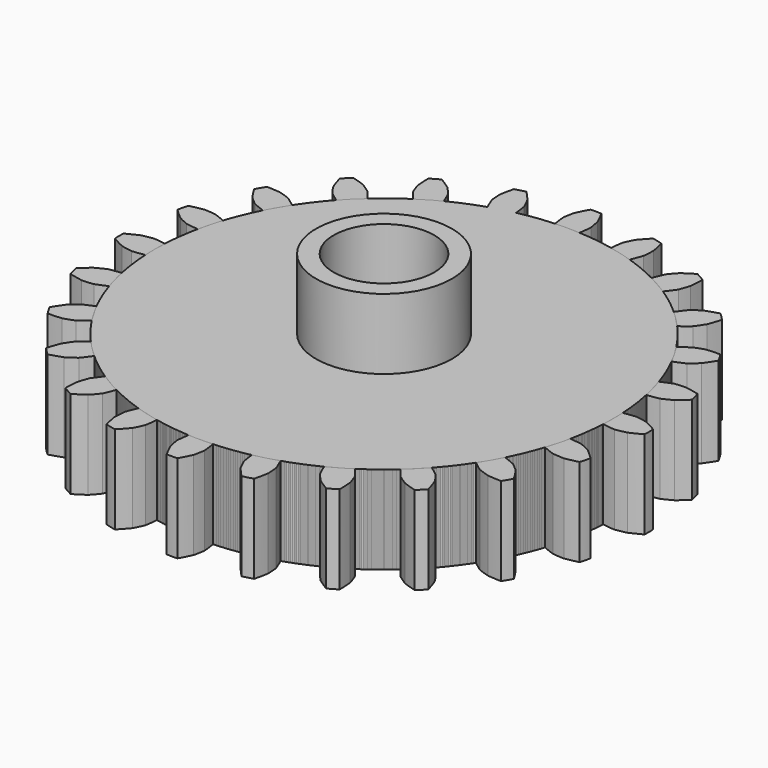
from build123d import *

# Parameters (mm, degrees)
F1_DEPTH = 5
F2_COUNT = 24
F3_R     = 2.85
F4_DEPTH = 25
F5_R     = 3.85
F5_R_2   = 2.85
F6_DEPTH = 4


# Not quite as in the source:
# - a feature of the source that left no trace in its solid (it failed there, or was rolled back) is left out


with BuildPart() as f1:
    # F0 (on Top) → F1 (new body)
    with BuildSketch(Plane.XY):
        with BuildLine():
            ThreePointArc((-0.6884619994, 12.9817572029), (-8.9456691759, -9.4326562005), (13, 0))
            ThreePointArc((13, 0), (9.4359199575, 8.9422264876), (0.6979362223, 12.9812512891))
            Line((0.6979362223, 12.9812512891), (0.6595878513, 12.8166601062))
            Line((0.6595878513, 12.8166601062), (-0.6884619994, 12.8166601062))
            Line((-0.6884619994, 12.8166601062), (-0.6884619994, 12.9817572029))
        make_face()
        with BuildLine():
            Line((0.6595878513, 12.8166601062), (0.6979362223, 12.9812512891))
            ThreePointArc((0.6979362223, 12.9812512891), (0.0047438605, 12.9999991345), (-0.6884619994, 12.9817572029))
            Line((-0.6884619994, 12.9817572029), (-0.6884619994, 12.8166601062))
            Line((-0.6884619994, 12.8166601062), (0.6595878513, 12.8166601062))
        make_face()
        with BuildLine():
            ThreePointArc((-0.6884619994, 12.9817572029), (0.0047438605, 12.9999991345), (0.6979362223, 12.9812512891))
            Line((0.6979362223, 12.9812512891), (0.7013501859, 12.9959040186))
            ThreePointArc((0.7013501859, 12.9959040186), (0.7485258682, 13.3381143086), (0.7812866085, 13.6820040604))
            ThreePointArc((0.7812866085, 13.6820040604), (0.7246476562, 14.0030111675), (0.6551136173, 14.3214739615))
            ThreePointArc((0.6551136173, 14.3214739615), (0.4878270863, 14.6723504286), (0.3076734335, 15.0167974346))
            ThreePointArc((0.3076734335, 15.0167974346), (0.0022476478, 15.0264990738), (-0.3031776772, 15.0167829421))
            ThreePointArc((-0.3031776772, 15.0167829421), (-0.4904903849, 14.6709788581), (-0.6630231094, 14.3175683689))
            ThreePointArc((-0.6630231094, 14.3175683689), (-0.7323663603, 14.0016121807), (-0.7822406896, 13.6820040604))
            ThreePointArc((-0.7822406896, 13.6820040604), (-0.7420135102, 13.3383984362), (-0.6884619994, 12.9966159225))
            Line((-0.6884619994, 12.9966159225), (-0.6884619994, 12.9817572029))
        make_face()
    extrude(amount=F1_DEPTH)


with BuildPart() as f2_1:
    # F2: instance of F1
    add(f1.part.rotate(Axis((0, 0, 0), (0, 0, -1)), 1 * 360 / F2_COUNT))


with BuildPart() as f2_2:
    # F2: instance of F1
    add(f1.part.rotate(Axis((0, 0, 0), (0, 0, -1)), 2 * 360 / F2_COUNT))


with BuildPart() as f2_3:
    # F2: instance of F1
    add(f1.part.rotate(Axis((0, 0, 0), (0, 0, -1)), 3 * 360 / F2_COUNT))


with BuildPart() as f2_4:
    # F2: instance of F1
    add(f1.part.rotate(Axis((0, 0, 0), (0, 0, -1)), 4 * 360 / F2_COUNT))


with BuildPart() as f2_5:
    # F2: instance of F1
    add(f1.part.rotate(Axis((0, 0, 0), (0, 0, -1)), 5 * 360 / F2_COUNT))


with BuildPart() as f2_6:
    # F2: instance of F1
    add(f1.part.rotate(Axis((0, 0, 0), (0, 0, -1)), 6 * 360 / F2_COUNT))


with BuildPart() as f2_7:
    # F2: instance of F1
    add(f1.part.rotate(Axis((0, 0, 0), (0, 0, -1)), 7 * 360 / F2_COUNT))


with BuildPart() as f2_8:
    # F2: instance of F1
    add(f1.part.rotate(Axis((0, 0, 0), (0, 0, -1)), 8 * 360 / F2_COUNT))


with BuildPart() as f2_9:
    # F2: instance of F1
    add(f1.part.rotate(Axis((0, 0, 0), (0, 0, -1)), 9 * 360 / F2_COUNT))


with BuildPart() as f2_10:
    # F2: instance of F1
    add(f1.part.rotate(Axis((0, 0, 0), (0, 0, -1)), 10 * 360 / F2_COUNT))


with BuildPart() as f2_11:
    # F2: instance of F1
    add(f1.part.rotate(Axis((0, 0, 0), (0, 0, -1)), 11 * 360 / F2_COUNT))


with BuildPart() as f2_12:
    # F2: instance of F1
    add(f1.part.rotate(Axis((0, 0, 0), (0, 0, -1)), 12 * 360 / F2_COUNT))


with BuildPart() as f2_13:
    # F2: instance of F1
    add(f1.part.rotate(Axis((0, 0, 0), (0, 0, -1)), 13 * 360 / F2_COUNT))


with BuildPart() as f2_14:
    # F2: instance of F1
    add(f1.part.rotate(Axis((0, 0, 0), (0, 0, -1)), 14 * 360 / F2_COUNT))


with BuildPart() as f2_15:
    # F2: instance of F1
    add(f1.part.rotate(Axis((0, 0, 0), (0, 0, -1)), 15 * 360 / F2_COUNT))


with BuildPart() as f2_16:
    # F2: instance of F1
    add(f1.part.rotate(Axis((0, 0, 0), (0, 0, -1)), 16 * 360 / F2_COUNT))


with BuildPart() as f2_17:
    # F2: instance of F1
    add(f1.part.rotate(Axis((0, 0, 0), (0, 0, -1)), 17 * 360 / F2_COUNT))


with BuildPart() as f2_18:
    # F2: instance of F1
    add(f1.part.rotate(Axis((0, 0, 0), (0, 0, -1)), 18 * 360 / F2_COUNT))


with BuildPart() as f2_19:
    # F2: instance of F1
    add(f1.part.rotate(Axis((0, 0, 0), (0, 0, -1)), 19 * 360 / F2_COUNT))


with BuildPart() as f2_20:
    # F2: instance of F1
    add(f1.part.rotate(Axis((0, 0, 0), (0, 0, -1)), 20 * 360 / F2_COUNT))


with BuildPart() as f2_21:
    # F2: instance of F1
    add(f1.part.rotate(Axis((0, 0, 0), (0, 0, -1)), 21 * 360 / F2_COUNT))


with BuildPart() as f2_22:
    # F2: instance of F1
    add(f1.part.rotate(Axis((0, 0, 0), (0, 0, -1)), 22 * 360 / F2_COUNT))


with BuildPart() as f2_23:
    # F2: instance of F1
    add(f1.part.rotate(Axis((0, 0, 0), (0, 0, -1)), 23 * 360 / F2_COUNT))


with BuildPart() as f4_tool:
    # F3 (on face) → F4 (new body)
    with BuildSketch(Plane.XY.offset(5)):
        Circle(F3_R)
    extrude(amount=-F4_DEPTH)


with BuildPart() as f1_1:
    add(f1.part)

    # F4: cut by f4_tool
    add(f4_tool.part, mode=Mode.SUBTRACT)


with BuildPart() as f2_1_1:
    add(f2_1.part)

    # F4: cut by f4_tool
    add(f4_tool.part, mode=Mode.SUBTRACT)


with BuildPart() as f2_2_1:
    add(f2_2.part)

    # F4: cut by f4_tool
    add(f4_tool.part, mode=Mode.SUBTRACT)


with BuildPart() as f2_3_1:
    add(f2_3.part)

    # F4: cut by f4_tool
    add(f4_tool.part, mode=Mode.SUBTRACT)


with BuildPart() as f2_4_1:
    add(f2_4.part)

    # F4: cut by f4_tool
    add(f4_tool.part, mode=Mode.SUBTRACT)


with BuildPart() as f2_5_1:
    add(f2_5.part)

    # F4: cut by f4_tool
    add(f4_tool.part, mode=Mode.SUBTRACT)


with BuildPart() as f2_6_1:
    add(f2_6.part)

    # F4: cut by f4_tool
    add(f4_tool.part, mode=Mode.SUBTRACT)


with BuildPart() as f2_7_1:
    add(f2_7.part)

    # F4: cut by f4_tool
    add(f4_tool.part, mode=Mode.SUBTRACT)


with BuildPart() as f2_8_1:
    add(f2_8.part)

    # F4: cut by f4_tool
    add(f4_tool.part, mode=Mode.SUBTRACT)


with BuildPart() as f2_9_1:
    add(f2_9.part)

    # F4: cut by f4_tool
    add(f4_tool.part, mode=Mode.SUBTRACT)


with BuildPart() as f2_10_1:
    add(f2_10.part)

    # F4: cut by f4_tool
    add(f4_tool.part, mode=Mode.SUBTRACT)


with BuildPart() as f2_11_1:
    add(f2_11.part)

    # F4: cut by f4_tool
    add(f4_tool.part, mode=Mode.SUBTRACT)


with BuildPart() as f2_12_1:
    add(f2_12.part)

    # F4: cut by f4_tool
    add(f4_tool.part, mode=Mode.SUBTRACT)


with BuildPart() as f2_13_1:
    add(f2_13.part)

    # F4: cut by f4_tool
    add(f4_tool.part, mode=Mode.SUBTRACT)


with BuildPart() as f2_14_1:
    add(f2_14.part)

    # F4: cut by f4_tool
    add(f4_tool.part, mode=Mode.SUBTRACT)


with BuildPart() as f2_15_1:
    add(f2_15.part)

    # F4: cut by f4_tool
    add(f4_tool.part, mode=Mode.SUBTRACT)


with BuildPart() as f2_16_1:
    add(f2_16.part)

    # F4: cut by f4_tool
    add(f4_tool.part, mode=Mode.SUBTRACT)


with BuildPart() as f2_17_1:
    add(f2_17.part)

    # F4: cut by f4_tool
    add(f4_tool.part, mode=Mode.SUBTRACT)


with BuildPart() as f2_18_1:
    add(f2_18.part)

    # F4: cut by f4_tool
    add(f4_tool.part, mode=Mode.SUBTRACT)


with BuildPart() as f2_19_1:
    add(f2_19.part)

    # F4: cut by f4_tool
    add(f4_tool.part, mode=Mode.SUBTRACT)


with BuildPart() as f2_20_1:
    add(f2_20.part)

    # F4: cut by f4_tool
    add(f4_tool.part, mode=Mode.SUBTRACT)


with BuildPart() as f2_21_1:
    add(f2_21.part)

    # F4: cut by f4_tool
    add(f4_tool.part, mode=Mode.SUBTRACT)


with BuildPart() as f2_22_1:
    add(f2_22.part)

    # F4: cut by f4_tool
    add(f4_tool.part, mode=Mode.SUBTRACT)


with BuildPart() as f2_23_1:
    add(f2_23.part)

    # F4: cut by f4_tool
    add(f4_tool.part, mode=Mode.SUBTRACT)


with BuildPart() as f6:
    # F5 (on face) → F6 (new body)
    with BuildSketch(Plane.XY.offset(5)):
        Circle(F5_R)
        Circle(F5_R_2, mode=Mode.SUBTRACT)
    extrude(amount=F6_DEPTH)


solid = Compound([f1_1.part, f2_1_1.part, f2_2_1.part, f2_3_1.part, f2_4_1.part, f2_5_1.part, f2_6_1.part, f2_7_1.part, f2_8_1.part, f2_9_1.part, f2_10_1.part, f2_11_1.part, f2_12_1.part, f2_13_1.part, f2_14_1.part, f2_15_1.part, f2_16_1.part, f2_17_1.part, f2_18_1.part, f2_19_1.part, f2_20_1.part, f2_21_1.part, f2_22_1.part, f2_23_1.part, f6.part])
